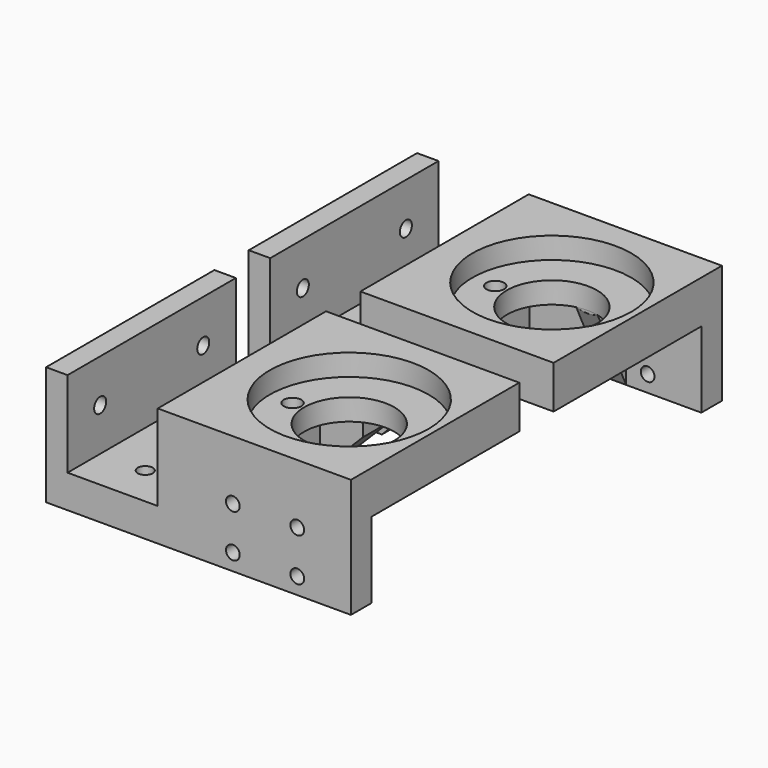
from build123d import *

# Parameters (mm, degrees)
F0_W      = 40
F0_H      = 27.7
F1_DEPTH  = 6
F2_W      = 40
F2_H      = 10
F3_DEPTH  = 43
F4_R      = 18.5
F5_DEPTH  = 5
F6_R      = 10.5
F6_R_2    = 2.05
F7_DEPTH  = 22.701
F8_W      = 43
F8_H      = 17.7
F9_DEPTH  = 31
F10_W     = 21
F10_H     = 20
F11_DEPTH = 49.001
F13_DEPTH = 17.7
F15_DEPTH = 5
F16_W     = 8
F16_H     = 17.7
F17_DEPTH = 10
F18_R     = 1.75
F19_DEPTH = 7.701
F20_R     = 1.75
F21_DEPTH = 5.001
F23_D     = 3.2
F24_SIZE  = 10


# Not quite as in the source:
# - a feature names something its author has since deleted; it is built from what else it names


with BuildPart() as f1:
    # F0 (on Front) → F1 (new body)
    with BuildSketch(Plane.XZ):
        with Locations((13.5, 13.85)):
            Rectangle(F0_W, F0_H)
    extrude(amount=F1_DEPTH)

    # F2 (on face) → F3 (join)
    with BuildSketch(Plane.XZ.offset(6)):
        with Locations((13.5, 22.7)):
            Rectangle(F2_W, F2_H)
    extrude(amount=F3_DEPTH)

    # F4 (on face) → F5 (cut)
    with BuildSketch(Plane.XY.offset(27.7)):
        with Locations((13.5, -24.5)):
            Circle(F4_R)
    extrude(amount=-F5_DEPTH, mode=Mode.SUBTRACT)

    # F6 (on face) → F7 (cut, through all)
    with BuildSketch(Plane.XY.offset(22.7)):
        with Locations((13.5, -24.5)):
            Circle(F6_R)
        with Locations((26.7, -24.5)):
            Circle(F6_R_2)
        with Locations((0.3, -24.5)):
            Circle(F6_R_2)
    extrude(amount=-F7_DEPTH, mode=Mode.SUBTRACT)

    # F8 (on face) → F9 (join)
    with BuildSketch(Plane(origin=(-6.5, 0, 0), x_dir=(0, -1, 0), z_dir=(-1, 0, 0))):
        Polygon((0, 27.7), (0, 0), (6, 0), (6, 17.7), (49, 17.7), (49, 27.7), align=None)
        with Locations((27.5, 8.85)):
            Rectangle(F8_W, F8_H)
    extrude(amount=F9_DEPTH)

    # F10 (on face) → F11 (cut, through all)
    with BuildSketch(Plane.XZ.offset(49)):
        with Locations((-22, 17.7)):
            Rectangle(F10_W, F10_H)
    extrude(amount=-F11_DEPTH, mode=Mode.SUBTRACT)

    # F12 (on face) → F13 (join, through all)
    with BuildSketch(Plane(origin=(0, 0, 17.7), x_dir=(1, 0, 0), z_dir=(0, 0, -1))):
        with BuildLine():
            Line((11, 14.3019609728), (11, 6))
            Line((11, 6), (16, 6))
            Line((16, 6), (16, 14.3019609728))
            ThreePointArc((16, 14.3019609728), (13.5, 14), (11, 14.3019609728))
        make_face()
    extrude(amount=F13_DEPTH)

    # F14 (on face) → F15 (cut, through all)
    with BuildSketch(Plane.YZ.offset(16)):
        Polygon((-6, 0), (-14.3019609728, 17.7), (-14.3019609728, 0), align=None)
    extrude(amount=-F15_DEPTH, mode=Mode.SUBTRACT)

    # F16 (on face) → F17 (join)
    with BuildSketch(Plane.YZ.offset(-6.5)):
        with Locations((-45, 8.85)):
            Rectangle(F16_W, F16_H)
    extrude(amount=F17_DEPTH)

    # F18 (on face) → F19 (cut, through all)
    with BuildSketch(Plane.XY.offset(7.7)):
        with Locations((-22, -39.5)):
            Circle(F18_R)
        with Locations((-22, -9.5)):
            Circle(F18_R)
    extrude(amount=-F19_DEPTH, mode=Mode.SUBTRACT)

    # F20 (on face) → F21 (cut, through all)
    with BuildSketch(Plane.YZ.offset(-32.5)):
        with Locations((-39.5, 17.7)):
            Circle(F20_R)
        with Locations((-9.5, 17.7)):
            Circle(F20_R)
    extrude(amount=-F21_DEPTH, mode=Mode.SUBTRACT)

    # F23 (through all)
    with Locations(Plane.XZ.offset(6)):
        with Locations((6, 3.85), (6, 13.85), (21, 13.85), (21, 3.85)):
            Hole(F23_D / 2)

    # F24
    f24_edges = [f1.edges().sort_by_distance(p)[0] for p in [
        (3.5, -45, 0),
    ]]
    chamfer(f24_edges, length=F24_SIZE)


with BuildPart() as f26_1:
    # F26: instance of F1
    add(f1.part.mirror(Plane(origin=(-4.6859618239, -54, 15.4693779987), x_dir=(1, 0, 0), z_dir=(0, -1, 0))))


solid = Compound([f1.part, f26_1.part])
